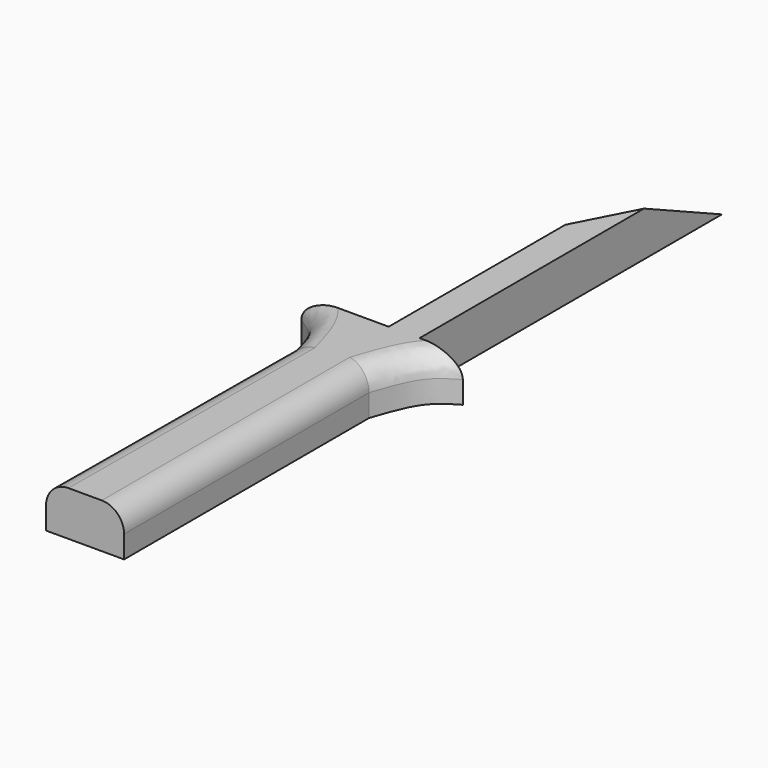
from build123d import *

# Parameters (mm, degrees)
F1_DEPTH = 5.08
F2_SIZE  = 5.07999
F3_R     = 2.54


# Not quite as in the source:
# - a fillet or chamfer is up to 0.001 mm smaller than in the source, because OpenCascade refuses the exact size


with BuildPart() as f1:
    # F0 (on Top) → F1 (new body)
    with BuildSketch(Plane.XY):
        Polygon((-50.5690909922, 21.4745439589), (-59.1589100659, 21.4745439589), (-59.2091714259, 13.8599455538), (-59.4360008836, -20.5047279596), (-50.5690909922, -20.5047279596), (-50.5690909922, 14.3012451008), align=None)
        with BuildLine():
            Line((-59.2091714259, 13.8599455538), (-59.1589100659, 21.4745439589))
            Line((-59.1589100659, 21.4745439589), (-64.0080049634, 21.4745439589))
            add(Edge.make_bspline(
                [(-64.0080049634, 21.4745439589), (-63.0207799447, 20.8576332232), (-60.7789769957, 19.4567445904), (-59.7724519982, 15.8681994581), (-59.2091714259, 13.8599455538)],
                knots=[0, 0, 0, 0, 0.4403710055, 1, 1, 1, 1], degree=3))
        make_face()
        Polygon((-59.1589100659, 47.79817909), (-59.1589100659, 21.4745439589), (-50.5690909922, 21.4745439589), (-50.5690909922, 64.423635602), align=None)
        with BuildLine():
            Line((-45.6602349877, 21.4745439589), (-50.5690909922, 21.4745439589))
            Line((-50.5690909922, 21.4745439589), (-50.5690909922, 14.3012451008))
            add(Edge.make_bspline(
                [(-45.6602349877, 21.4745439589), (-46.6065278441, 20.9184128466), (-48.770914008, 19.6464149903), (-49.9215342609, 16.2261394646), (-50.5690909922, 14.3012451008)],
                knots=[0, 0, 0, 0, 0.4372107307, 1, 1, 1, 1], degree=3))
        make_face()
    extrude(amount=F1_DEPTH)

    # F2 (size 5.08 in the source; OpenCascade refuses exactly that, so slightly less here)
    f2_edges = [f1.edges().sort_by_distance(p)[0] for p in [
        (-59.15891, 34.636362, 5.08),
        (-54.864001, 56.110907, 5.08),
    ]]
    chamfer(f2_edges, length=F2_SIZE)

    # F3
    f3_edges = [f1.edges().sort_by_distance(p)[0] for p in [
        (-59.322586, -3.322391, 5.08),
        (-50.569091, -3.101741, 5.08),
        (-60.725717, 18.263642, 5.08),
        (-48.908594, 18.46974, 5.08),
    ]]
    fillet(f3_edges, radius=F3_R)


solid = f1.part
